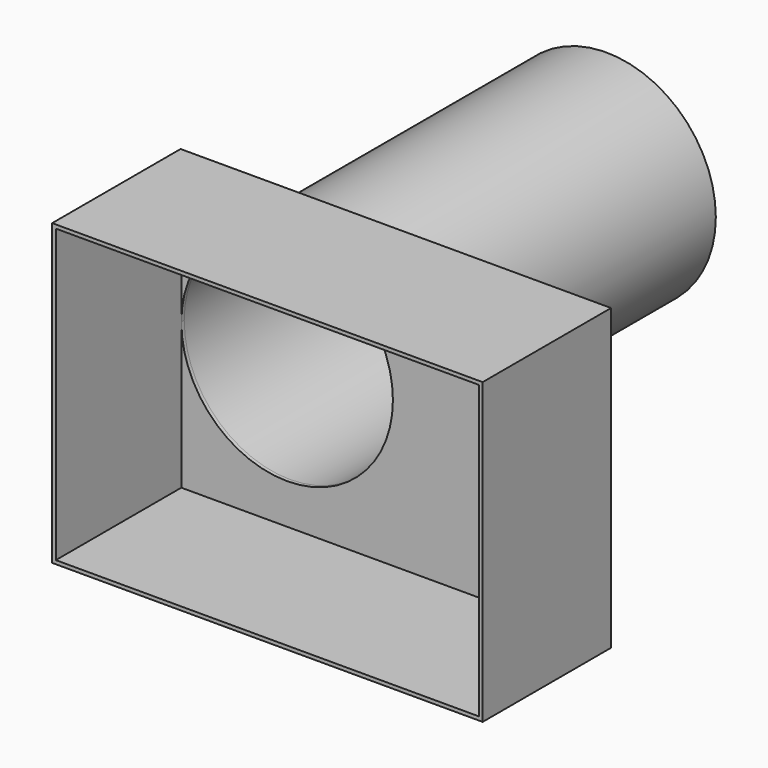
from build123d import *

# Parameters (mm, degrees)
F0_W        = 59
F0_H        = 41
F1_DEPTH    = 22
F2_R        = 15
F3_DEPTH    = 76.2
F4_T        = 0.5
F4_T4_ANGLE = 180.000000001
F4_T6_ANGLE = 180.000000001


# Not quite as in the source:
# - a shell that OpenCascade refuses in one call is made with other operations: the cavity is built on its own and cut out


with BuildPart() as f1:
    # F0 (on Front) → F1 (new body)
    with BuildSketch(Plane.XZ):
        Rectangle(F0_W, F0_H)
    extrude(amount=-F1_DEPTH)

    # F2 (on Front) → F3 (join)
    with BuildSketch(Plane.XZ):
        with Locations((-14.5, 0)):
            Circle(F2_R)
    extrude(amount=-F3_DEPTH)

    # F4: shell of thickness 0.5, made by hand


with BuildPart() as f4_core1:
    # F4_t2: copy of F1
    add(f1.part)

    # the walls: a layer under each face that stays
    f4_faces = [f4_core1.faces().sort_by_distance(p)[0] for p in [
        (29.5, 11, 0),
        (0, 22, -13.6666666667),
        (-29.5, 49.1, 0),
        (-14.5, 76.2, 0),
        (-29.5, 11, 0),
        (0, 11, 20.5),
        (0, 11, -20.5),
    ]]
    thicken(f4_faces, amount=-F4_T, mode=Mode.SUBTRACT)

    # F4_s3 → F4_t4 (revolve, cut)
    with BuildSketch(Plane.XY):
        Polygon((-29.505, 22.005), (-29.5, 21.5), (-29, 21.5), (-29, 22), align=None)
    revolve(axis=Axis((-14.5, 22, 0), (0, -1, 0)), revolution_arc=F4_T4_ANGLE, mode=Mode.SUBTRACT)

    # F4_s5 → F4_t6 (revolve, cut)
    with BuildSketch(Plane.XY):
        Polygon((0.505, 22.005), (0.5, 21.5), (0, 21.5), (0, 22), align=None)
    revolve(axis=Axis((-14.5, 22, 0), (0, -1, 0)), revolution_arc=F4_T6_ANGLE, mode=Mode.SUBTRACT)


with BuildPart() as f1_1:
    add(f1.part)

    # what is left inside the walls is the cavity
    f4_cavity = [f4_core1.part.solids().sort_by_distance(p)[0] for p in [
        (-28.995, 57.8, 0),
    ]]
    add(f4_cavity, mode=Mode.SUBTRACT)


solid = f1_1.part
